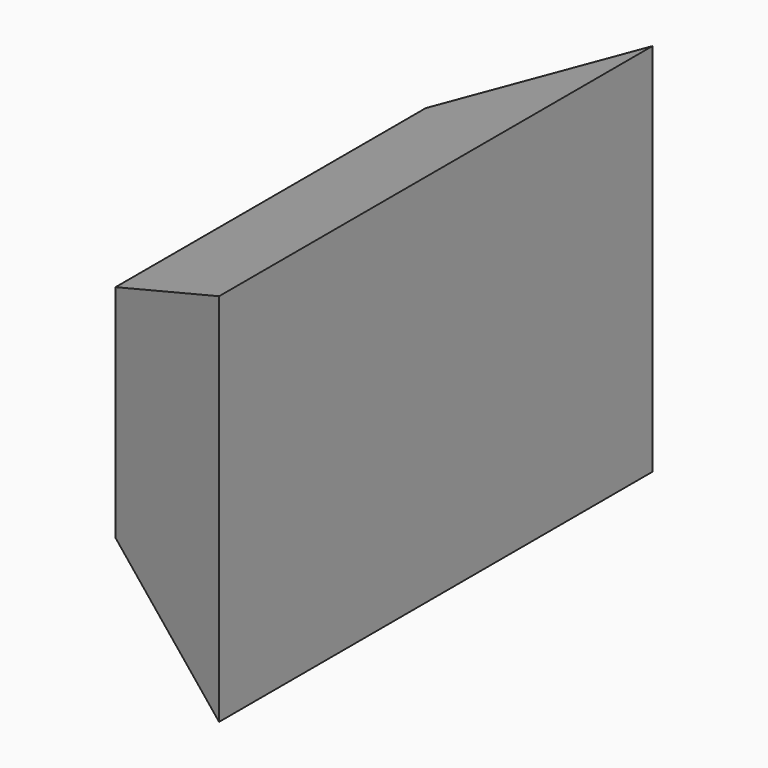
from build123d import *

# Parameters (mm, degrees)
F0_W     = 234.8122149706
F0_H     = 133.6912661791
F1_DEPTH = 100
F1_TAPER = -25


with BuildPart() as f1:
    # F0 (on Right) → F1 (new body)
    with BuildSketch(Plane.YZ):
        Rectangle(F0_W, F0_H)
    extrude(amount=F1_DEPTH, taper=F1_TAPER)


solid = f1.part
